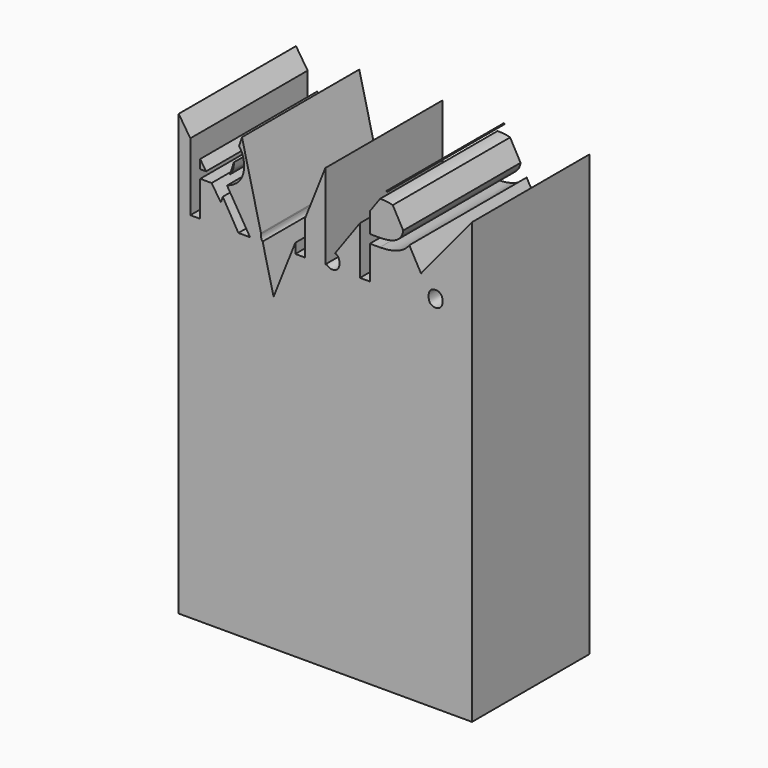
from build123d import *

# Parameters (mm, degrees)
F1_DEPTH     = 12.7
F2_TEXT_SIZE = 10.2802188353
F3_DEPTH     = 25.4


# Not quite as in the source:
# - Text() gives the source's letters only with a copy of the font that has no kerning and outlines rounded to 1/6400 em; it was checked with that copy


with BuildPart() as f1:
    # F0 (on Front) → F1 (new body)
    with BuildSketch(Plane.XZ):
        Polygon((-12.7, 48.6465214424), (-12.7, 10.5465214424), (12.7, 10.5465214424), (12.7, 48.6465214424), (8.2852365449, 43.2968735695), (5.3210752085, 48.6465214424), (0, 41.244763881), (0, 48.6465214424), (-4.4834623113, 37.3685508966), (-7.2196130641, 48.6465214424), (-9.0437121689, 43.0688634515), align=None)
    extrude(amount=F1_DEPTH)

    # F2 (on face) → F3 (cut)
    with BuildSketch(Plane.XZ.offset(12.7)):
        with Locations((-12.7, 41.244763881)):
            Text('R.I.P.', F2_TEXT_SIZE, font='Open Sans', text_align=(TextAlign.LEFT, TextAlign.BOTTOM))
    extrude(amount=-F3_DEPTH, mode=Mode.SUBTRACT)


solid = f1.part
